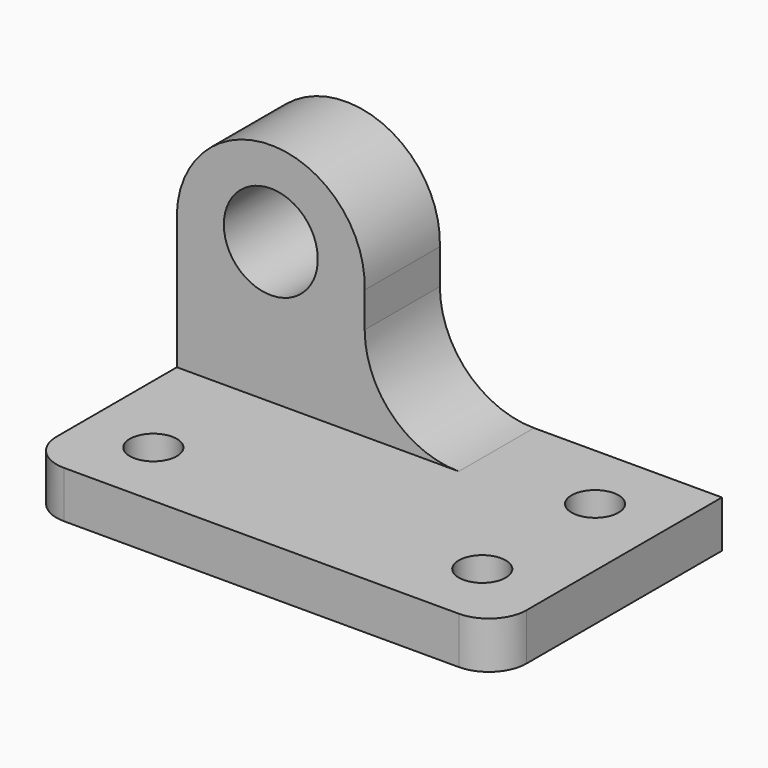
from build123d import *

# Parameters (mm, degrees)
F2_DEPTH  = 38.1
F3_W      = 25.4
F3_H      = 31.75
F4_DEPTH  = 25.4
F5_DEPTH  = 12.7
F7_D      = 12.7
F9_DEPTH  = 12.7
F10_DEPTH = 123
F11_R     = 5.08
F13_D     = 6.35
F15_D     = 6.35
F17_D     = 6.35


# Not quite as in the source:
# - an extrude ends at something that could not be found from the text; its depth is read off the source's solid


with BuildPart() as f2:
    # F0 (on Front) → F2 (new body)
    with BuildSketch(Plane.XZ):
        Polygon((-15.0914756011, 53.4695235106), (-53.1914756011, 53.4695235106), (-53.1914756011, 15.3695235106), (10.3085243989, 15.3695235106), (10.3085243989, 21.7195235106), (-15.0914756011, 21.7195235106), align=None)
    extrude(amount=F2_DEPTH)

    # F3 (on face) → F4 (cut)
    with BuildSketch(Plane.YZ.offset(-15.0914756011)):
        with Locations((-25.4, 37.5945235106)):
            Rectangle(F3_W, F3_H)
    extrude(amount=-F4_DEPTH, mode=Mode.SUBTRACT)

    # F5 (cut): a face of the model
    f5_faces = [f2.faces().sort_by_distance(p)[0] for p in [
        (-40.4914756011, -25.4, 37.5945235106),
    ]]
    extrude(f5_faces, amount=-F5_DEPTH, mode=Mode.SUBTRACT)

    # F7 (through all)
    with Locations(Plane.XZ.offset(12.7)):
        with Locations((-40.4914756011, 40.7695235106)):
            Hole(F7_D / 2)

    # F8 (on face) → F9 (cut)
    with BuildSketch(Plane.XZ.offset(12.7)):
        with BuildLine():
            ThreePointArc((-53.1914756011, 40.0317125094), (-40.0621213537, 52.2842661721), (-27.8065160195, 39.1577604642))
            Line((-27.8065160195, 39.1577604642), (-27.8065160195, 34.4195235106))
            ThreePointArc((-27.8065160195, 34.4195235106), (-24.0770508865, 25.4383560684), (-15.0914756011, 21.7195235106))
            Line((-15.0914756011, 21.7195235106), (-15.0914756011, 53.4695235106))
            Line((-15.0914756011, 53.4695235106), (-53.1914756011, 53.4695235106))
            Line((-53.1914756011, 53.4695235106), (-53.1914756011, 40.0317125094))
        make_face()
    extrude(amount=-F9_DEPTH, mode=Mode.SUBTRACT)

    # F1 (on face) → F10 (cut, through all)
    with BuildSketch(Plane.XZ):
        Polygon((-15.0914756011, 21.7195235106), (-15.0914756011, 53.4695235106), (-53.1914756011, 53.4695235106), (-53.1914756011, 15.3695235106), (10.3085243989, 15.3695235106), (10.3085243989, 21.7195235106), align=None)
    extrude(amount=-F10_DEPTH, mode=Mode.SUBTRACT)

    # F11
    f11_edges = [f2.edges().sort_by_distance(p)[0] for p in [
        (-53.191476, -38.1, 18.544524),
        (10.308524, -38.1, 18.544524),
    ]]
    fillet(f11_edges, radius=F11_R)

    # F13 (through all)
    with Locations(Plane.XY.offset(21.7195235106)):
        with Locations((-43.6664756011, -28.575)):
            Hole(F13_D / 2)

    # F15 (through all)
    with Locations(Plane.XY.offset(21.7195235106)):
        with Locations((0.7835243989, -9.525)):
            Hole(F15_D / 2)

    # F17 (through all)
    with Locations(Plane.XY.offset(21.7195235106)):
        with Locations((0.7835243989, -28.575)):
            Hole(F17_D / 2)


solid = f2.part
